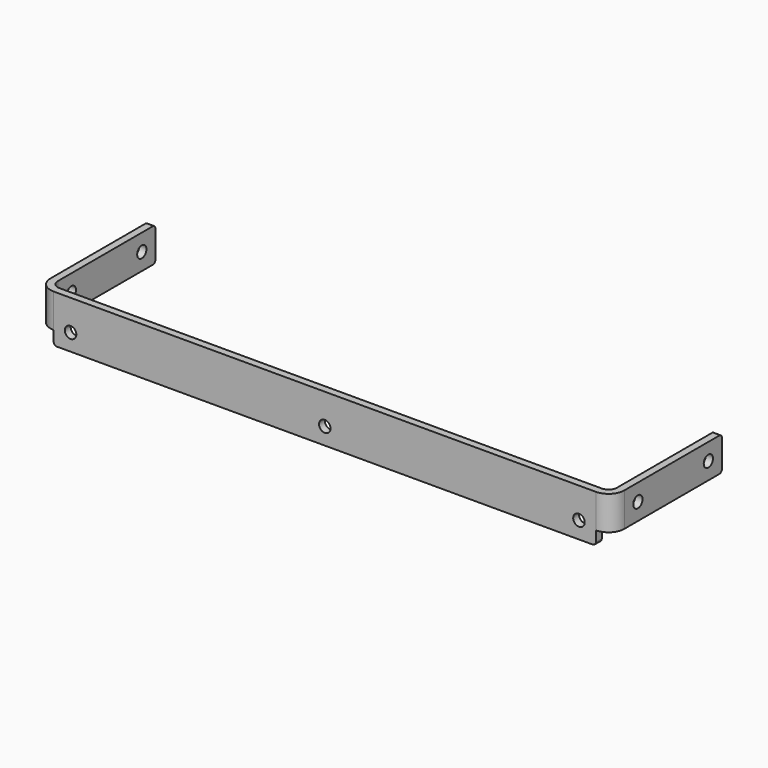
from build123d import *

# Parameters (mm, degrees)
F1_DEPTH = 7.9375
F2_R     = 1.98374
F3_R     = 3.69316
F4_R     = 1.35255
F5_DEPTH = 134.38632
F6_W     = 127
F6_H     = 1.70942
F7_DEPTH = 3.175
F8_R     = 1.35255
F9_DEPTH = 1.70942
F10_R    = 0.762


with BuildPart() as f1:
    # F0 (on Top) → F1 (new body)
    with BuildSketch(Plane.XY):
        Polygon((0, 30.55874), (0, 0), (-130.96748, 0), (-130.96748, 30.55874), (-132.6769, 30.55874), (-132.6769, -1.70942), (1.70942, -1.70942), (1.70942, 30.55874), align=None)
    extrude(amount=F1_DEPTH)

    # F2
    f2_edges = [f1.edges().sort_by_distance(p)[0] for p in [
        (0, 0, 3.96875),
        (-130.96748, 0, 3.96875),
    ]]
    fillet(f2_edges, radius=F2_R)

    # F3
    f3_edges = [f1.edges().sort_by_distance(p)[0] for p in [
        (1.70942, -1.70942, 3.96875),
        (-132.6769, -1.70942, 3.96875),
    ]]
    fillet(f3_edges, radius=F3_R)

    # F4 (on face) → F5 (cut, through all)
    with BuildSketch(Plane(origin=(-132.6769, 0, 0), x_dir=(0, -1, 0), z_dir=(-1, 0, 0))):
        with Locations((-26.58999, 3.96875)):
            Circle(F4_R)
        with Locations((-5.95249, 3.96875)):
            Circle(F4_R)
    extrude(amount=-F5_DEPTH, mode=Mode.SUBTRACT)

    # F6 (on face) → F7 (join)
    with BuildSketch(Plane(origin=(0, 0, 0), x_dir=(1, 0, 0), z_dir=(0, 0, -1))):
        with Locations((-65.48374, 0.85471)):
            Rectangle(F6_W, F6_H)
    extrude(amount=F7_DEPTH)

    # F8 (on face) → F9 (cut, through all)
    with BuildSketch(Plane.XZ.offset(1.70942)):
        with Locations((-125.01499, 0.79375)):
            Circle(F8_R)
        with Locations((-65.48374, 0.79375)):
            Circle(F8_R)
        with Locations((-5.95249, 0.79375)):
            Circle(F8_R)
    extrude(amount=-F9_DEPTH, mode=Mode.SUBTRACT)

    # F10
    f10_edges = [f1.edges().sort_by_distance(p)[0] for p in [
        (0.85471, 30.55874, 0),
        (0.85471, 30.55874, 7.9375),
        (-131.82219, 30.55874, 0),
        (-131.82219, 30.55874, 7.9375),
        (-128.98374, -0.85471, -3.175),
        (-1.98374, -0.85471, -3.175),
    ]]
    fillet(f10_edges, radius=F10_R)


solid = f1.part
